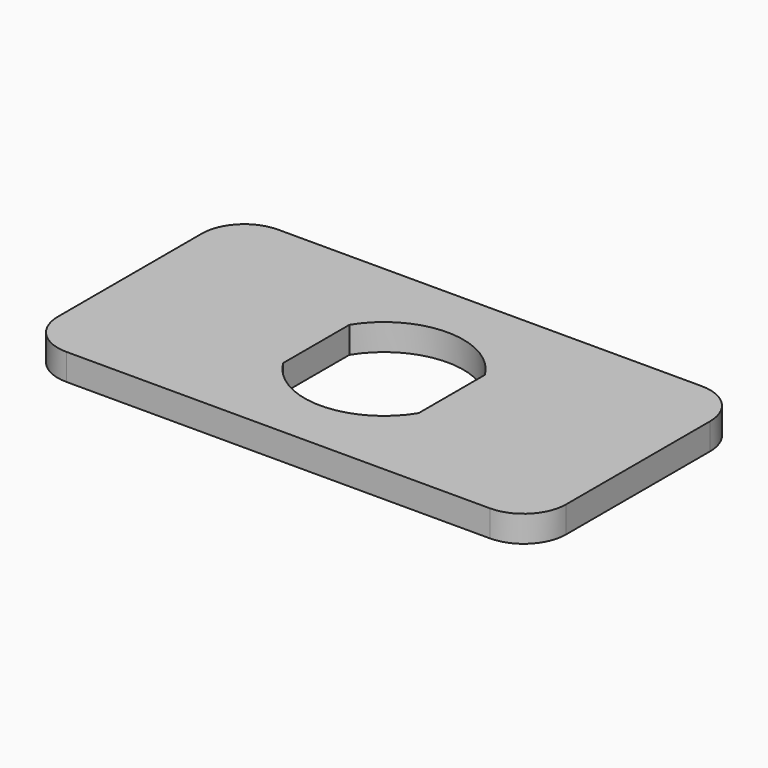
from build123d import *

# Parameters (mm, degrees)
F0_W     = 60.96
F0_H     = 31.75
F1_DEPTH = 3.175
F2_R     = 5.08


# Not quite as in the source:
# - a length typed as a fraction of an inch, garbled in the dataset ("3 / 203.2 mm" for 3/8 in), is restored


with BuildPart() as f1:
    # F0 (on Top) → F1 (new body)
    with BuildSketch(Plane.XY):
        Rectangle(F0_W, F0_H)
        with BuildLine():
            Line((-8.128, -4.9660085582), (-8.128, 4.9660085582))
            ThreePointArc((-8.128, 4.9660085582), (0, 9.525), (8.128, 4.9660085582))
            Line((8.128, 4.9660085582), (8.128, -4.9660085582))
            ThreePointArc((8.128, -4.9660085582), (0, -9.525), (-8.128, -4.9660085582))
        make_face(mode=Mode.SUBTRACT)
    extrude(amount=F1_DEPTH)

    # F2
    f2_edges = [f1.edges().sort_by_distance(p)[0] for p in [
        (-30.48, 15.875, 1.5875),
        (30.48, 15.875, 1.5875),
        (-30.48, -15.875, 1.5875),
        (30.48, -15.875, 1.5875),
    ]]
    fillet(f2_edges, radius=F2_R)


solid = f1.part
